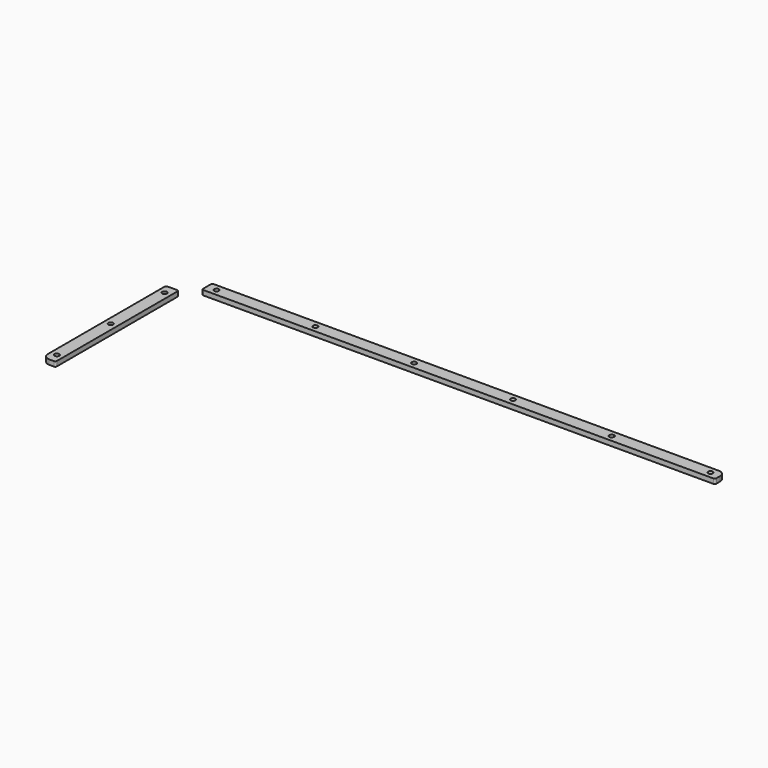
from build123d import *

# Parameters (mm, degrees)
F0_R     = 2.38125
F1_DEPTH = 4.7625
F4_W     = 148.8558202982
F4_H     = 38.4750810385
F4_W_2   = 12.7
F4_H_2   = 12.7
F5_DEPTH = 4.7635
F7_DEPTH = 4.7625


# Not quite as in the source:
# - a feature of the source that left no trace in its solid (it failed there, or was rolled back) is left out


with BuildPart() as f1:
    # F0 (on Top) → F1 (new body)
    with BuildSketch(Plane.XY):
        with BuildLine():
            ThreePointArc((0, 6.35), (1.8598719395, 1.8598719395), (6.35, 0))
            Line((6.35, 0), (527.05, 0))
            ThreePointArc((527.05, 0), (531.5401280605, 1.8598719395), (533.4, 6.35))
            Line((533.4, 6.35), (533.4, 171.45))
            ThreePointArc((533.4, 171.45), (531.5401280605, 175.9401280605), (527.05, 177.8))
            Line((527.05, 177.8), (336.55, 177.8))
            ThreePointArc((336.55, 177.8), (332.0598719395, 179.6598719395), (330.2, 184.15))
            Line((330.2, 184.15), (330.2, 203.2))
            ThreePointArc((330.2, 203.2), (328.3401280605, 207.6901280605), (323.85, 209.55))
            Line((323.85, 209.55), (209.55, 209.55))
            ThreePointArc((209.55, 209.55), (205.0598719395, 207.6901280605), (203.2, 203.2))
            Line((203.2, 203.2), (203.2, 184.15))
            ThreePointArc((203.2, 184.15), (201.3401280605, 179.6598719395), (196.85, 177.8))
            Line((196.85, 177.8), (6.35, 177.8))
            ThreePointArc((6.35, 177.8), (1.8598719395, 175.9401280605), (0, 171.45))
            Line((0, 171.45), (0, 6.35))
        make_face()
        with Locations((6.35, 9.525)):
            Circle(F0_R, mode=Mode.SUBTRACT)
        with Locations((257.175, 30.1625)):
            Circle(F0_R, mode=Mode.SUBTRACT)
        with Locations((6.35, 76.2)):
            Circle(F0_R, mode=Mode.SUBTRACT)
        with Locations((257.175, 93.6625)):
            Circle(F0_R, mode=Mode.SUBTRACT)
        with Locations((485.775, 30.1625)):
            Circle(F0_R, mode=Mode.SUBTRACT)
        with Locations((485.775, 93.6625)):
            Circle(F0_R, mode=Mode.SUBTRACT)
        with Locations((6.35, 142.875)):
            Circle(F0_R, mode=Mode.SUBTRACT)
        with Locations((34.925, 171.45)):
            Circle(F0_R, mode=Mode.SUBTRACT)
        with Locations((132.715, 171.45)):
            Circle(F0_R, mode=Mode.SUBTRACT)
        with Locations((230.505, 171.45)):
            Circle(F0_R, mode=Mode.SUBTRACT)
        with Locations((223.8375, 195.2625)):
            Circle(F0_R, mode=Mode.SUBTRACT)
        with Locations((239.7125, 185.7375)):
            Circle(F0_R, mode=Mode.SUBTRACT)
        with Locations((328.295, 171.45)):
            Circle(F0_R, mode=Mode.SUBTRACT)
        with Locations((293.6875, 185.7375)):
            Circle(F0_R, mode=Mode.SUBTRACT)
        with Locations((309.5625, 195.2625)):
            Circle(F0_R, mode=Mode.SUBTRACT)
        with Locations((426.085, 171.45)):
            Circle(F0_R, mode=Mode.SUBTRACT)
        with Locations((523.875, 171.45)):
            Circle(F0_R, mode=Mode.SUBTRACT)
    extrude(amount=F1_DEPTH)

    # F4 (on face) → F5 (cut, through all)
    with BuildSketch(Plane.XY.offset(4.7625)):
        with Locations((269.9074968696, 197.0375405192)):
            Rectangle(F4_W, F4_H)
        Polygon((25.4, 185.5913083792), (-12.6593864247, 185.5913083792), (-12.6593864247, 152.4), (12.7, 152.4), (12.7, 165.1), (25.4, 165.1), align=None)
        Polygon((533.4, 165.1), (25.4, 165.1), (25.4, 152.4), (12.7, 152.4), (12.7, 0), (533.4, 0), align=None)
        with Locations((19.05, 158.75)):
            Rectangle(F4_W_2, F4_H_2)
    extrude(amount=-F5_DEPTH, mode=Mode.SUBTRACT)

    # F6 (on face) → F7 (cut, through all)
    with BuildSketch(Plane.XY.offset(4.7625)):
        with BuildLine():
            Line((12.7, 150.8125), (12.7, 152.4))
            Line((12.7, 152.4), (11.1125, 152.4))
            ThreePointArc((11.1125, 152.4), (12.2350320151, 151.9350320151), (12.7, 150.8125))
        make_face()
        with BuildLine():
            Line((1.5875, 152.4), (0, 152.4))
            Line((0, 152.4), (0, 150.8125))
            ThreePointArc((0, 150.8125), (0.4649679849, 151.9350320151), (1.5875, 152.4))
        make_face()
        with BuildLine():
            ThreePointArc((12.7, 1.5875), (12.2350320151, 0.4649679849), (11.1125, 0))
            Line((11.1125, 0), (12.7, 0))
            Line((12.7, 0), (12.7, 1.5875))
        make_face()
        with BuildLine():
            ThreePointArc((25.4, 176.2125), (25.8649679849, 177.3350320151), (26.9875, 177.8))
            Line((26.9875, 177.8), (25.4, 177.8))
            Line((25.4, 177.8), (25.4, 176.2125))
        make_face()
        with BuildLine():
            ThreePointArc((26.9875, 165.1), (25.8649679849, 165.5649679849), (25.4, 166.6875))
            Line((25.4, 166.6875), (25.4, 165.1))
            Line((25.4, 165.1), (26.9875, 165.1))
        make_face()
        with BuildLine():
            ThreePointArc((533.4, 166.6875), (532.9350320151, 165.5649679849), (531.8125, 165.1))
            Line((531.8125, 165.1), (533.4, 165.1))
            Line((533.4, 165.1), (533.4, 166.6875))
        make_face()
    extrude(amount=-F7_DEPTH, mode=Mode.SUBTRACT)


solid = f1.part
